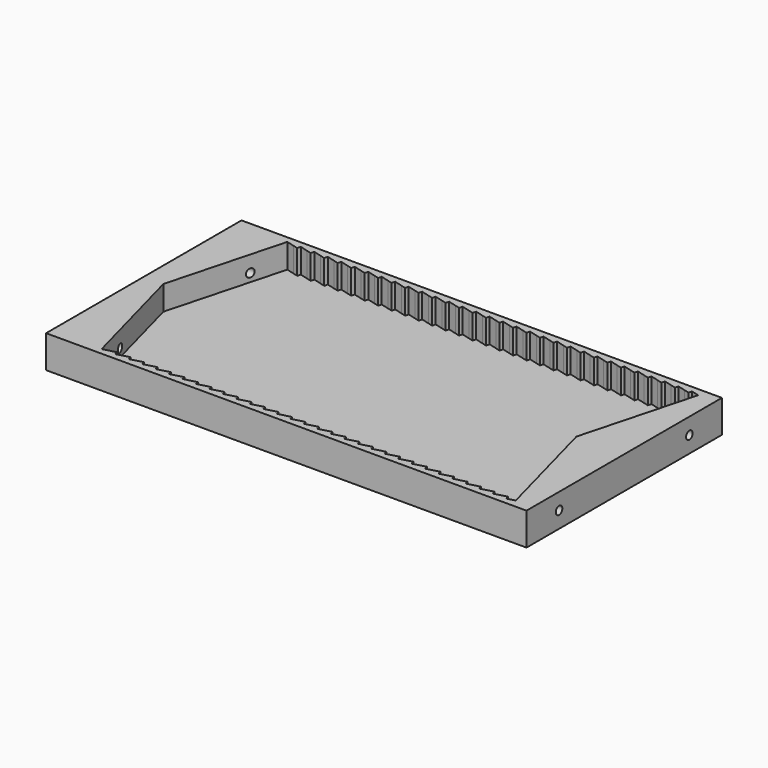
from build123d import *

# Parameters (mm, degrees)
F0_W     = 295
F0_H     = 150
F1_DEPTH = 20
F3_D     = 5
F6_DEPTH = 15


# Not quite as in the source:
# - ends of sketch curves that miss each other by under 0.0002 mm in the source are joined
# - a feature names something its author has since deleted; it is built from what else it names


with BuildPart() as f1:
    # F0 (on Top) → F1 (new body)
    with BuildSketch(Plane.XY):
        Rectangle(F0_W, F0_H)
    extrude(amount=F1_DEPTH)

    # F3 (through all)
    with Locations(Plane.YZ.offset(147.5)):
        with Locations((-50, 10), (50, 10)):
            Hole(F3_D / 2)

    # F5 (on face) → F6 (cut)
    with BuildSketch(Plane.XY.offset(20)):
        Polygon((-116.396805, 71.294095), (-135.5, 0), (-116.396805, -71.294095), (-111.567176, -70), (-130.323619, 0), (-111.567176, 70), align=None)
        Polygon((-108.669398, 69.223543), (-111.567176, 70), (-130.323619, 0), (-111.567176, -70), (-108.669398, -69.223543), (-127.217791, 0), align=None)
        Polygon((-108.114595, 71.294095), (-108.669398, 69.223543), (-127.217791, 0), (-108.669398, -69.223543), (-108.114595, -71.294095), (-103.284966, -70), (-122.041409, 0), (-103.284966, 70), align=None)
        Polygon((-100.387188, 69.223543), (-103.284966, 70), (-122.041409, 0), (-103.284966, -70), (-100.387188, -69.223543), (-118.935581, 0), align=None)
        Polygon((-99.832385, 71.294095), (-100.387188, 69.223543), (-118.935581, 0), (-100.387188, -69.223543), (-99.832385, -71.294095), (-95.002756, -70), (-113.759199, 0), (-95.002756, 70), align=None)
        Polygon((-92.104978, 69.223543), (-95.002756, 70), (-113.759199, 0), (-95.002756, -70), (-92.104978, -69.223543), (-110.653371, 0), align=None)
        Polygon((-91.550175, 71.294095), (-92.104978, 69.223543), (-110.653371, 0), (-92.104978, -69.223543), (-91.550175, -71.294095), (-86.720546, -70), (-105.476989, 0), (-86.720546, 70), align=None)
        Polygon((-83.822768, 69.223543), (-86.720546, 70), (-105.476989, 0), (-86.720546, -70), (-83.822768, -69.223543), (-102.371161, 0), align=None)
        Polygon((-83.267965, 71.294095), (-83.822768, 69.223543), (-102.371161, 0), (-83.822768, -69.223543), (-83.267965, -71.294095), (-78.438336, -70), (-97.194779, 0), (-78.438336, 70), align=None)
        Polygon((-75.540558, 69.223543), (-78.438336, 70), (-97.194779, 0), (-78.438336, -70), (-75.540558, -69.223543), (-94.088951, 0), align=None)
        Polygon((-74.985755, 71.294095), (-75.540558, 69.223543), (-94.088951, 0), (-75.540558, -69.223543), (-74.985755, -71.294095), (-70.156126, -70), (-88.912569, 0), (-70.156126, 70), align=None)
        Polygon((-67.258348, 69.223543), (-70.156126, 70), (-88.912569, 0), (-70.156126, -70), (-67.258348, -69.223543), (-85.806741, 0), align=None)
        Polygon((-66.703545, 71.294095), (-67.258348, 69.223543), (-85.806741, 0), (-67.258348, -69.223543), (-66.703545, -71.294095), (-61.873916, -70), (-80.630359, 0), (-61.873916, 70), align=None)
        Polygon((-58.976138, 69.223543), (-61.873916, 70), (-80.630359, 0), (-61.873916, -70), (-58.976138, -69.223543), (-77.524531, 0), align=None)
        Polygon((-58.421335, 71.294095), (-58.976138, 69.223543), (-77.524531, 0), (-58.976138, -69.223543), (-58.421335, -71.294095), (-53.591706, -70), (-72.348149, 0), (-53.591706, 70), align=None)
        Polygon((-50.693928, 69.223543), (-53.591706, 70), (-72.348149, 0), (-53.591706, -70), (-50.693928, -69.223543), (-69.242321, 0), align=None)
        Polygon((-50.139125, 71.294095), (-50.693928, 69.223543), (-69.242321, 0), (-50.693928, -69.223543), (-50.139125, -71.294095), (-45.309496, -70), (-64.065939, 0), (-45.309496, 70), align=None)
        Polygon((-42.411718, 69.223543), (-45.309496, 70), (-64.065939, 0), (-45.309496, -70), (-42.411718, -69.223543), (-60.960111, 0), align=None)
        Polygon((-41.856915, 71.294095), (-42.411718, 69.223543), (-60.960111, 0), (-42.411718, -69.223543), (-41.856915, -71.294095), (-37.027286, -70), (-55.783729, 0), (-37.027286, 70), align=None)
        Polygon((-34.129508, 69.223543), (-37.027286, 70), (-55.783729, 0), (-37.027286, -70), (-34.129508, -69.223543), (-52.677901, 0), align=None)
        Polygon((-33.574705, 71.294095), (-34.129508, 69.223543), (-52.677901, 0), (-34.129508, -69.223543), (-33.574705, -71.294095), (-28.745076, -70), (-47.501519, 0), (-28.745076, 70), align=None)
        Polygon((-25.847298, 69.223543), (-28.745076, 70), (-47.501519, 0), (-28.745076, -70), (-25.847298, -69.223543), (-44.395691, 0), align=None)
        Polygon((-25.292495, 71.294095), (-25.847298, 69.223543), (-44.395691, 0), (-25.847298, -69.223543), (-25.292495, -71.294095), (-20.462866, -70), (-39.219309, 0), (-20.462866, 70), align=None)
        Polygon((-17.565088, 69.223543), (-20.462866, 70), (-39.219309, 0), (-20.462866, -70), (-17.565088, -69.223543), (-36.113481, 0), align=None)
        Polygon((-17.010285, 71.294095), (-17.565088, 69.223543), (-36.113481, 0), (-17.565088, -69.223543), (-17.010285, -71.294095), (-12.180656, -70), (-30.937099, 0), (-12.180656, 70), align=None)
        Polygon((-9.282878, 69.223543), (-12.180656, 70), (-30.937099, 0), (-12.180656, -70), (-9.282878, -69.223543), (-27.831271, 0), align=None)
        Polygon((-8.728075, 71.294095), (-9.282878, 69.223543), (-27.831271, 0), (-9.282878, -69.223543), (-8.728075, -71.294095), (-3.898446, -70), (-22.654889, 0), (-3.898446, 70), align=None)
        Polygon((-1.000668, 69.223543), (-3.898446, 70), (-22.654889, 0), (-3.898446, -70), (-1.000668, -69.223543), (-19.549061, 0), align=None)
        Polygon((-0.445865, 71.294095), (-1.000668, 69.223543), (-19.549061, 0), (-1.000668, -69.223543), (-0.445865, -71.294095), (4.383764, -70), (-14.372679, 0), (4.383764, 70), align=None)
        Polygon((7.281542, 69.223543), (4.383764, 70), (-14.372679, 0), (4.383764, -70), (7.281542, -69.223543), (-11.266851, 0), align=None)
        Polygon((7.836345, 71.294095), (7.281542, 69.223543), (-11.266851, 0), (7.281542, -69.223543), (7.836345, -71.294095), (12.665974, -70), (-6.090469, 0), (12.665974, 70), align=None)
        Polygon((15.563752, 69.223543), (12.665974, 70), (-6.090469, 0), (12.665974, -70), (15.563752, -69.223543), (-2.984641, 0), align=None)
        Polygon((16.118555, 71.294095), (15.563752, 69.223543), (-2.984641, 0), (15.563752, -69.223543), (16.118555, -71.294095), (20.948184, -70), (2.191741, 0), (20.948184, 70), align=None)
        Polygon((23.845962, 69.223543), (20.948184, 70), (2.191741, 0), (20.948184, -70), (23.845962, -69.223543), (5.297569, 0), align=None)
        Polygon((24.400765, 71.294095), (23.845962, 69.223543), (5.297569, 0), (23.845962, -69.223543), (24.400765, -71.294095), (29.230394, -70), (10.473951, 0), (29.230394, 70), align=None)
        Polygon((32.128172, 69.223543), (29.230394, 70), (10.473951, 0), (29.230394, -70), (32.128172, -69.223543), (13.579779, 0), align=None)
        Polygon((32.682975, 71.294095), (32.128172, 69.223543), (13.579779, 0), (32.128172, -69.223543), (32.682975, -71.294095), (37.512604, -70), (18.756161, 0), (37.512604, 70), align=None)
        Polygon((40.410382, 69.223543), (37.512604, 70), (18.756161, 0), (37.512604, -70), (40.410382, -69.223543), (21.861989, 0), align=None)
        Polygon((40.965185, 71.294095), (40.410382, 69.223543), (21.861989, 0), (40.410382, -69.223543), (40.965185, -71.294095), (45.794814, -70), (27.038371, 0), (45.794814, 70), align=None)
        Polygon((48.692592, 69.223543), (45.794814, 70), (27.038371, 0), (45.794814, -70), (48.692592, -69.223543), (30.144199, 0), align=None)
        Polygon((49.247395, 71.294095), (48.692592, 69.223543), (30.144199, 0), (48.692592, -69.223543), (49.247395, -71.294095), (54.077024, -70), (35.320581, 0), (54.077024, 70), align=None)
        Polygon((56.974802, 69.223543), (54.077024, 70), (35.320581, 0), (54.077024, -70), (56.974802, -69.223543), (38.426409, 0), align=None)
        Polygon((57.529605, 71.294095), (56.974802, 69.223543), (38.426409, 0), (56.974802, -69.223543), (57.529605, -71.294095), (62.359234, -70), (43.602791, 0), (62.359234, 70), align=None)
        Polygon((65.257012, 69.223543), (62.359234, 70), (43.602791, 0), (62.359234, -70), (65.257012, -69.223543), (46.708619, 0), align=None)
        Polygon((65.811815, 71.294095), (65.257012, 69.223543), (46.708619, 0), (65.257012, -69.223543), (65.811815, -71.294095), (70.641444, -70), (51.885001, 0), (70.641444, 70), align=None)
        Polygon((73.539222, 69.223543), (70.641444, 70), (51.885001, 0), (70.641444, -70), (73.539222, -69.223543), (54.990829, 0), align=None)
        Polygon((74.094025, 71.294095), (73.539222, 69.223543), (54.990829, 0), (73.539222, -69.223543), (74.094025, -71.294095), (78.923654, -70), (60.167211, 0), (78.923654, 70), align=None)
        Polygon((81.821432, 69.223543), (78.923654, 70), (60.167211, 0), (78.923654, -70), (81.821432, -69.223543), (63.273039, 0), align=None)
        Polygon((82.376235, 71.294095), (81.821432, 69.223543), (63.273039, 0), (81.821432, -69.223543), (82.376235, -71.294095), (87.205864, -70), (68.449421, 0), (87.205864, 70), align=None)
        Polygon((90.103642, 69.223543), (87.205864, 70), (68.449421, 0), (87.205864, -70), (90.103642, -69.223543), (71.555249, 0), align=None)
        Polygon((90.658445, 71.294095), (90.103642, 69.223543), (71.555249, 0), (90.103642, -69.223543), (90.658445, -71.294095), (95.488074, -70), (76.731631, 0), (95.488074, 70), align=None)
        Polygon((98.385852, 69.223543), (95.488074, 70), (76.731631, 0), (95.488074, -70), (98.385852, -69.223543), (79.837459, 0), align=None)
        Polygon((98.940655, 71.294095), (98.385852, 69.223543), (79.837459, 0), (98.385852, -69.223543), (98.940655, -71.294095), (103.770284, -70), (85.013841, 0), (103.770284, 70), align=None)
        Polygon((106.668062, 69.223543), (103.770284, 70), (85.013841, 0), (103.770284, -70), (106.668062, -69.223543), (88.119669, 0), align=None)
        Polygon((107.222865, 71.294095), (106.668062, 69.223543), (88.119669, 0), (106.668062, -69.223543), (107.222865, -71.294095), (112.052494, -70), (93.296051, 0), (112.052494, 70), align=None)
        Polygon((114.950272, 69.223543), (112.052494, 70), (93.296051, 0), (112.052494, -70), (114.950272, -69.223543), (96.401879, 0), align=None)
        Polygon((115.505075, 71.294095), (114.950272, 69.223543), (96.401879, 0), (114.950272, -69.223543), (115.505075, -71.294095), (120.334704, -70), (101.578261, 0), (120.334704, 70), align=None)
        Polygon((123.232482, 69.223543), (120.334704, 70), (101.578261, 0), (120.334704, -70), (123.232482, -69.223543), (104.684089, 0), align=None)
        Polygon((123.787285, 71.294095), (123.232482, 69.223543), (104.684089, 0), (123.232482, -69.223543), (123.787285, -71.294095), (128.616914, -70), (109.860471, 0), (128.616914, 70), align=None)
        Polygon((131.514692, 69.223543), (128.616914, 70), (109.860471, 0), (128.616914, -70), (131.514692, -69.223543), (112.966299, 0), align=None)
        Polygon((132.069495, 71.294095), (131.514692, 69.223543), (112.966299, 0), (131.514692, -69.223543), (132.069495, -71.294095), (136.899124, -70), (118.14268, 0), (136.899124, 70), align=None)
    extrude(amount=-F6_DEPTH, mode=Mode.SUBTRACT)


solid = f1.part
